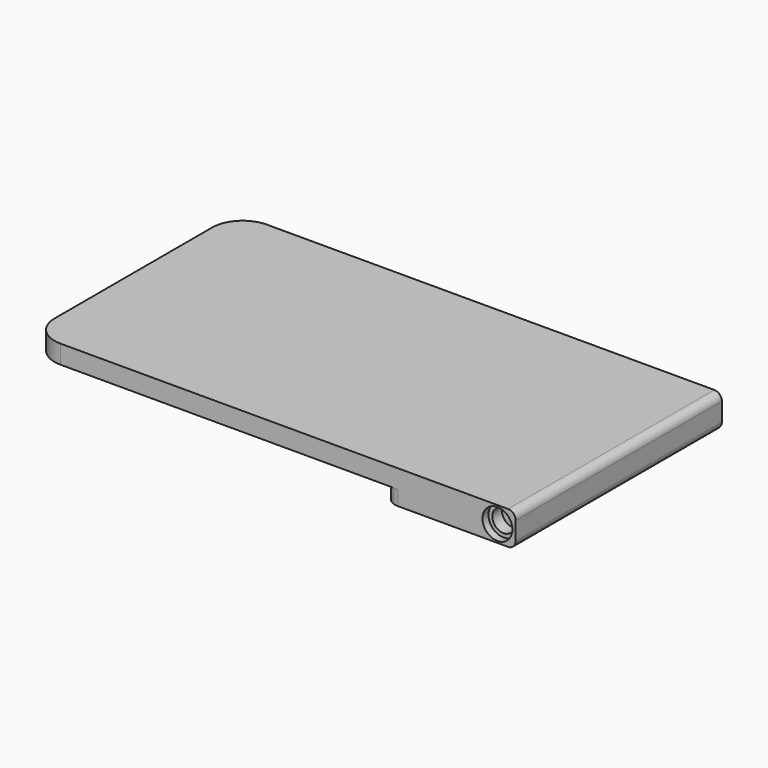
from build123d import *

# Parameters (mm, degrees)
F1_DEPTH = 4.4
F3_DEPTH = 1.95
F6_R     = 1.475
F8_DEPTH = 2.6
F6_R_2   = 1.975
F9_DEPTH = 1
F10_R    = 1


# Not quite as in the source:
# - a pattern or mirror of a feature is missing from the dataset's text; its kind, count and spacing are read off the source's solid


with BuildPart() as f1:
    # F0 (on Top) → F1 (new body)
    with BuildSketch(Plane.XY):
        with BuildLine():
            Line((-60, 0), (0, 0))
            Line((0, 0), (0, 34))
            Line((0, 34), (-60, 34))
            ThreePointArc((-60, 34), (-62.8284271247, 32.8284271247), (-64, 30))
            Line((-64, 30), (-64, 4))
            ThreePointArc((-64, 4), (-62.8284271247, 1.1715728753), (-60, 0))
        make_face()
    extrude(amount=F1_DEPTH)

    # F2 (on face) → F3 (cut)
    with BuildSketch(Plane(origin=(0, 0, 0), x_dir=(1, 0, 0), z_dir=(0, 0, -1))):
        with BuildLine():
            ThreePointArc((-15.5, -34), (-16.9142135624, -33.4142135624), (-17.5, -32))
            Line((-17.5, -32), (-17.5, -30.5))
            ThreePointArc((-17.5, -30.5), (-16.9142135624, -29.0857864376), (-15.5, -28.5))
            Line((-15.5, -28.5), (-4, -28.5))
            Line((-4, -28.5), (-4, -5.5))
            Line((-4, -5.5), (-15.5, -5.5))
            ThreePointArc((-15.5, -5.5), (-16.9142135624, -4.9142135624), (-17.5, -3.5))
            Line((-17.5, -3.5), (-17.5, -2))
            ThreePointArc((-17.5, -2), (-16.9142135624, -0.5857864376), (-15.5, 0))
            Line((-15.5, 0), (-64, 0))
            Line((-64, 0), (-64, -34))
            Line((-64, -34), (-15.5, -34))
        make_face()
    extrude(amount=-F3_DEPTH, mode=Mode.SUBTRACT)

    # F6 (on face) → F8 (cut)
    with BuildSketch(Plane.XZ):
        with Locations((-2.4, 2.2)):
            Circle(F6_R)
    f8 = extrude(amount=-F8_DEPTH, mode=Mode.SUBTRACT)

    # F8_copies: F8 across plane
    add(f8.mirror(Plane.ZX.offset(17)), mode=Mode.SUBTRACT)

    # F6 (on face) → F9 (cut)
    with BuildSketch(Plane.XZ):
        with Locations((-2.4, 2.2)):
            Circle(F6_R_2)
        with Locations((-2.4, 2.2)):
            Circle(F6_R, mode=Mode.SUBTRACT)
    f9 = extrude(amount=-F9_DEPTH, mode=Mode.SUBTRACT)

    # F9_copies: F9 across plane
    add(f9.mirror(Plane.ZX.offset(17)), mode=Mode.SUBTRACT)

    # F10
    f10_edges = [f1.edges().sort_by_distance(p)[0] for p in [
        (0, 17, 4.4),
        (0, 17, 0),
    ]]
    fillet(f10_edges, radius=F10_R)


solid = f1.part
